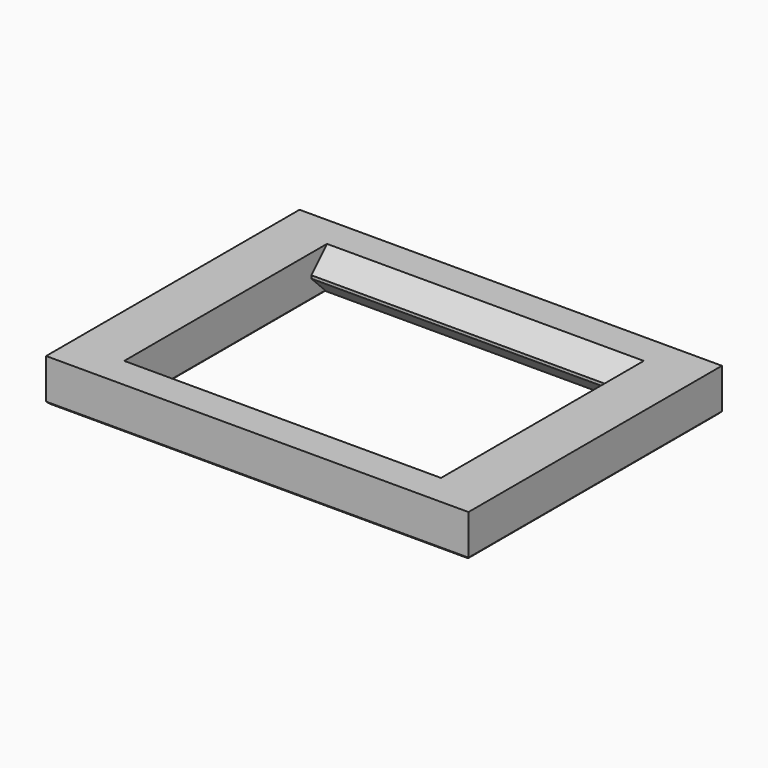
from build123d import *

# Parameters (mm, degrees)
F0_W         = 40
F0_H         = 30
F0_W_2       = 30
F0_H_2       = 24
F4_DEPTH     = 30
F5_SIZE      = 0.2
F6_T1_DEPTH  = 31.0286731952
F6_T3_DEPTH  = 41.0286731952
F6_T5_DEPTH  = 30
F6_T10_DEPTH = 25.0286731952
F6_T16_DEPTH = 25.0286731952
F6_T23_DEPTH = 25.0286731952
F6_T27_DEPTH = 30.225714172
F6_T34_DEPTH = 25.0286731952
F6_T38_DEPTH = 30.225714172
F6_T45_DEPTH = 30.225714172
F6_T49_DEPTH = 25.0286731952
F6_T56_DEPTH = 25.0286731952
F6_T60_DEPTH = 30.225714172


# Not quite as in the source:
# - a fillet or chamfer that OpenCascade refuses, or shapes differently, is made with other operations: its cross-section is extruded or revolved along the edge and cut away or added


with BuildPart() as f2:
    # F2: sweep along a path in F1
    with BuildLine(Plane.XZ) as f2_path:
        Line((0, 0), (0, -4))
    # F0 (on Top) → F2 (sweep)
    with BuildSketch(Plane.XY):
        Rectangle(F0_W, F0_H)
        Rectangle(F0_W_2, F0_H_2, mode=Mode.SUBTRACT)
    sweep(path=f2_path.line)

    # F3 (on face) → F4 (join, through all)
    with BuildSketch(Plane.YZ.offset(-15)):
        Polygon((-10, -2), (-12, 0), (-12, -4), align=None)
        Polygon((10, -2), (12, -4), (12, 0), align=None)
    extrude(amount=F4_DEPTH)

    # F5
    f5_edges = [f2.edges().sort_by_distance(p)[0] for p in [
        (0, -10, -2),
        (0, 10, -2),
    ]]
    chamfer(f5_edges, length=F5_SIZE)

    # F6: chamfer of 0.2 on 8 edges, made by hand

    # F6_s2 → F6_t1 (cut)
    with BuildSketch(Plane.XZ.offset(-15.5143365976)):
        Polygon((19.8, -4), (20, -3.8), (20, -4), align=None)
        Polygon((-19.8, -4), (-20, -3.8), (-20, -4), align=None)
    extrude(amount=F6_T1_DEPTH, mode=Mode.SUBTRACT)

    # F6_s4 → F6_t3 (cut)
    with BuildSketch(Plane.YZ.offset(-20.5143365976)):
        Polygon((-14.8, -4), (-15, -3.8), (-15, -4), align=None)
        Polygon((14.8, -4), (15, -3.8), (15, -4), align=None)
    extrude(amount=F6_T3_DEPTH, mode=Mode.SUBTRACT)

    # F6_s6 → F6_t5 (cut)
    with BuildSketch(Plane.YZ.offset(-15)):
        Polygon((-11.9414213562, -3.9414213562), (-12.0828427125, -4), (-12, -4), align=None)
        Polygon((12.0828427125, -4), (11.9414213562, -3.9414213562), (12, -4), align=None)
    extrude(amount=F6_T5_DEPTH, mode=Mode.SUBTRACT)


with BuildPart() as f6_tool8:
    # F6_s9 → F6_t10 (new body)
    with BuildSketch(Plane.XZ.offset(12.5143365976)):
        Polygon((-15, -3.8), (-15.2, -4), (-15, -4), align=None)
    extrude(amount=-F6_T10_DEPTH)

    split(bisect_by=Plane(origin=(0, -4, 4), x_dir=(1, 0, 0), z_dir=(0, 0.7071067812, -0.7071067812)), keep=Keep.TOP)

    split(bisect_by=Plane(origin=(0, 4, 4), x_dir=(1, 0, 0), z_dir=(0, -0.7071067812, -0.7071067812)), keep=Keep.TOP)


with BuildPart() as f2_1:
    add(f2.part)

    # F6_t7: cut F6_tool8
    add(f6_tool8.part, mode=Mode.SUBTRACT)


with BuildPart() as f6_tool14:
    # F6_s15 → F6_t16 (new body)
    with BuildSketch(Plane.XZ.offset(-12.5143365976)):
        Polygon((15.2, -4), (15, -3.8), (15, -4), align=None)
    extrude(amount=F6_T16_DEPTH)

    split(bisect_by=Plane(origin=(0, -4, 4), x_dir=(1, 0, 0), z_dir=(0, 0.7071067812, -0.7071067812)), keep=Keep.TOP)

    split(bisect_by=Plane(origin=(0, 4, 4), x_dir=(1, 0, 0), z_dir=(0, -0.7071067812, -0.7071067812)), keep=Keep.TOP)


with BuildPart() as f2_2:
    add(f2_1.part)

    # F6_t13: cut F6_tool14
    add(f6_tool14.part, mode=Mode.SUBTRACT)


with BuildPart() as f6_tool21:
    # F6_s22 → F6_t23 (new body)
    with BuildSketch(Plane.XZ.offset(12.5143365976)):
        Polygon((-15, -3.8), (-15.2, -4), (-15, -4), align=None)
    extrude(amount=-F6_T23_DEPTH)

    split(bisect_by=Plane(origin=(0, -4, 4), x_dir=(1, 0, 0), z_dir=(0, -0.7071067812, 0.7071067812)), keep=Keep.TOP)


with BuildPart() as f6_tool25:
    # F6_s26 → F6_t27 (new body)
    with BuildSketch(Plane.YZ.offset(15)):
        Polygon((-11.9414213562, -3.9414213562), (-12.0828427125, -4), (-12, -4), align=None)
    extrude(amount=-F6_T27_DEPTH)

    split(bisect_by=Plane.YZ.offset(-15), keep=Keep.BOTTOM)


with BuildPart() as f6_tool21_1:
    add(f6_tool21.part)

    # F6_t29: intersect F6_tool25
    add(f6_tool25.part, mode=Mode.INTERSECT)


with BuildPart() as f2_3:
    add(f2_2.part)

    # F6_t19: cut F6_tool21
    add(f6_tool21_1.part, mode=Mode.SUBTRACT)


with BuildPart() as f6_tool32:
    # F6_s33 → F6_t34 (new body)
    with BuildSketch(Plane.XZ.offset(12.5143365976)):
        Polygon((-15, -3.8), (-15.2, -4), (-15, -4), align=None)
    extrude(amount=-F6_T34_DEPTH)

    split(bisect_by=Plane(origin=(0, 4, 4), x_dir=(1, 0, 0), z_dir=(0, 0.7071067812, 0.7071067812)), keep=Keep.TOP)


with BuildPart() as f6_tool36:
    # F6_s37 → F6_t38 (new body)
    with BuildSketch(Plane.YZ.offset(-15.225714172)):
        Polygon((12.0828427125, -4), (11.9414213562, -3.9414213562), (12, -4), align=None)
    extrude(amount=F6_T38_DEPTH)

    split(bisect_by=Plane.YZ.offset(-15), keep=Keep.BOTTOM)


with BuildPart() as f6_tool32_1:
    add(f6_tool32.part)

    # F6_t40: intersect F6_tool36
    add(f6_tool36.part, mode=Mode.INTERSECT)


with BuildPart() as f2_4:
    add(f2_3.part)

    # F6_t30: cut F6_tool32
    add(f6_tool32_1.part, mode=Mode.SUBTRACT)


with BuildPart() as f6_tool43:
    # F6_s44 → F6_t45 (new body)
    with BuildSketch(Plane.YZ.offset(15.225714172)):
        Polygon((-11.9414213562, -3.9414213562), (-12.0828427125, -4), (-12, -4), align=None)
    extrude(amount=-F6_T45_DEPTH)

    split(bisect_by=Plane.YZ.offset(15), keep=Keep.TOP)


with BuildPart() as f6_tool47:
    # F6_s48 → F6_t49 (new body)
    with BuildSketch(Plane.XZ.offset(-12.5143365976)):
        Polygon((15.2, -4), (15, -3.8), (15, -4), align=None)
    extrude(amount=F6_T49_DEPTH)

    split(bisect_by=Plane(origin=(0, -4, 4), x_dir=(1, 0, 0), z_dir=(0, -0.7071067812, 0.7071067812)), keep=Keep.TOP)


with BuildPart() as f6_tool43_1:
    add(f6_tool43.part)

    # F6_t51: intersect F6_tool47
    add(f6_tool47.part, mode=Mode.INTERSECT)


with BuildPart() as f2_5:
    add(f2_4.part)

    # F6_t41: cut F6_tool43
    add(f6_tool43_1.part, mode=Mode.SUBTRACT)


with BuildPart() as f6_tool54:
    # F6_s55 → F6_t56 (new body)
    with BuildSketch(Plane.XZ.offset(-12.5143365976)):
        Polygon((15.2, -4), (15, -3.8), (15, -4), align=None)
    extrude(amount=F6_T56_DEPTH)

    split(bisect_by=Plane(origin=(0, 4, 4), x_dir=(1, 0, 0), z_dir=(0, 0.7071067812, 0.7071067812)), keep=Keep.TOP)


with BuildPart() as f6_tool58:
    # F6_s59 → F6_t60 (new body)
    with BuildSketch(Plane.YZ.offset(-15)):
        Polygon((12.0828427125, -4), (11.9414213562, -3.9414213562), (12, -4), align=None)
    extrude(amount=F6_T60_DEPTH)

    split(bisect_by=Plane.YZ.offset(15), keep=Keep.TOP)


with BuildPart() as f6_tool54_1:
    add(f6_tool54.part)

    # F6_t62: intersect F6_tool58
    add(f6_tool58.part, mode=Mode.INTERSECT)


with BuildPart() as f2_6:
    add(f2_5.part)

    # F6_t52: cut F6_tool54
    add(f6_tool54_1.part, mode=Mode.SUBTRACT)


solid = f2_6.part
